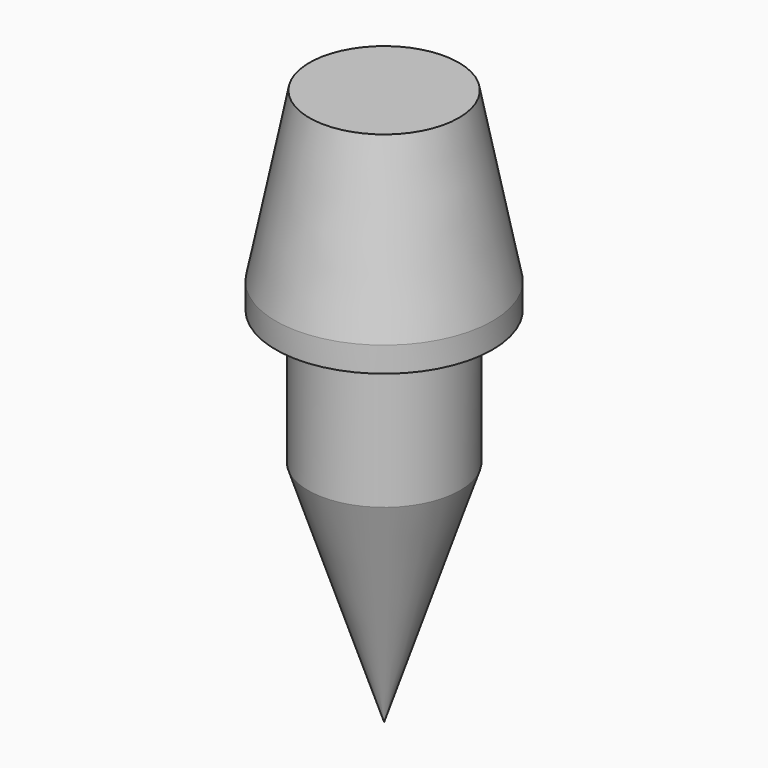
from build123d import *

# Parameters (mm, degrees)
F0_R     = 5.74675
F1_DEPTH = 10.16
F2_R     = 8.1915
F2_R_2   = 5.74675
F3_DEPTH = 1.905
F4_R     = 8.1915
F5_DEPTH = 12.7
F6_SIZE2 = 12.7
F6_SIZE  = 2.54
F7_DEPTH = 17.272
F8_SIZE2 = 5.74039
F8_SIZE  = 17.27199


# Not quite as in the source:
# - a fillet or chamfer is up to 0.001 mm smaller than in the source, because OpenCascade refuses the exact size


with BuildPart() as f1:
    # F0 (on Top) → F1 (new body)
    with BuildSketch(Plane.XY):
        Circle(F0_R)
    extrude(amount=F1_DEPTH)

    # F2 (on face) → F3 (join)
    with BuildSketch(Plane.XY.offset(10.16)):
        Circle(F2_R)
        Circle(F2_R_2, mode=Mode.SUBTRACT)
        Circle(F2_R_2)
    extrude(amount=F3_DEPTH)

    # F4 (on face) → F5 (join)
    with BuildSketch(Plane.XY.offset(12.065)):
        Circle(F4_R)
    extrude(amount=F5_DEPTH)

    # F6
    f6_edges = [f1.edges().sort_by_distance(p)[0] for p in [
        (-8.1915, 0, 24.765),
    ]]
    f6_side = f1.faces().sort_by_distance((0, 0, 24.765))[0]
    chamfer(f6_edges, length=F6_SIZE, length2=F6_SIZE2, reference=f6_side)

    # F7 (add): a face of the model
    f7_faces = [f1.faces().sort_by_distance(p)[0] for p in [
        (0, 0, 0),
    ]]
    extrude(f7_faces, amount=F7_DEPTH)

    # F8 (size 17.272 and 5.7404 in the source; OpenCascade refuses exactly that, so slightly less here)
    f8_edges = [f1.edges().sort_by_distance(p)[0] for p in [
        (-5.74675, 0, -17.272),
    ]]
    f8_side = f1.faces().sort_by_distance((-5.74675, 0, -8.636))[0]
    chamfer(f8_edges, length=F8_SIZE, length2=F8_SIZE2, reference=f8_side)


solid = f1.part
